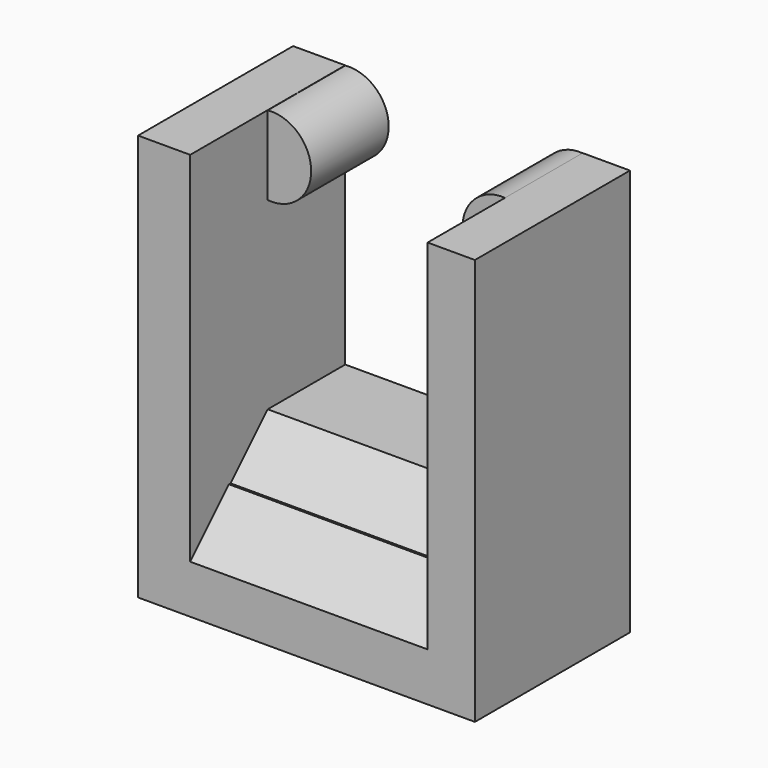
from build123d import *

# Parameters (mm, degrees)
F1_DEPTH    = 50.8
F2_R        = 10.405428205
F3_DEPTH    = 25.4
F4_T1_DEPTH = 62.2300039977
F5_W        = 88.3073359728
F5_H        = 50.8
F6_DEPTH    = 25.4
F7_SIZE     = 12.7


# Not quite as in the source:
# - a fillet or chamfer that OpenCascade refuses, or shapes differently, is made with other operations: its cross-section is extruded or revolved along the edge and cut away or added


with BuildPart() as f1:
    # F0 (on Front) → F1 (new body)
    with BuildSketch(Plane.XZ):
        Polygon((-31.2631689012, 40.7458357513), (-44.9346460508, 40.7458357513), (-44.9346460508, -40.4495000839), (43.372689922, -40.4495000839), (43.372689922, 40.7458357513), (30.9668350965, 40.7458357513), (30.9668350965, -28.2998345792), (-31.2631689012, -28.2998345792), align=None)
    extrude(amount=F1_DEPTH)

    # F2 (on Front) → F3 (join)
    with BuildSketch(Plane.XZ):
        with Locations((-30.2724801004, 30.3404075463)):
            Circle(F2_R)
        with Locations((30.2025526762, 30.3404075463)):
            Circle(F2_R)
    extrude(amount=F3_DEPTH)

    # F4: chamfer of 25.4 on 1 edges, made by hand

    # F4_s2 → F4_t1 (cut)
    with BuildSketch(Plane.YZ.offset(-31.2631689012)):
        Polygon((-50.8, -53.6998345792), (-25.4, -28.2998345792), (-50.8, -28.2998345792), align=None)
    extrude(amount=F4_T1_DEPTH, mode=Mode.SUBTRACT)

    # F5 (on face) → F6 (join)
    with BuildSketch(Plane(origin=(0, 0, -40.4495000839), x_dir=(1, 0, 0), z_dir=(0, 0, -1))):
        with Locations((-0.7809780644, 25.4)):
            Rectangle(F5_W, F5_H)
    extrude(amount=F6_DEPTH)

    # F7
    f7_edges = [f1.edges().sort_by_distance(p)[0] for p in [
        (-0.148167, -50.8, -40.4495),
    ]]
    chamfer(f7_edges, length=F7_SIZE)


solid = f1.part
